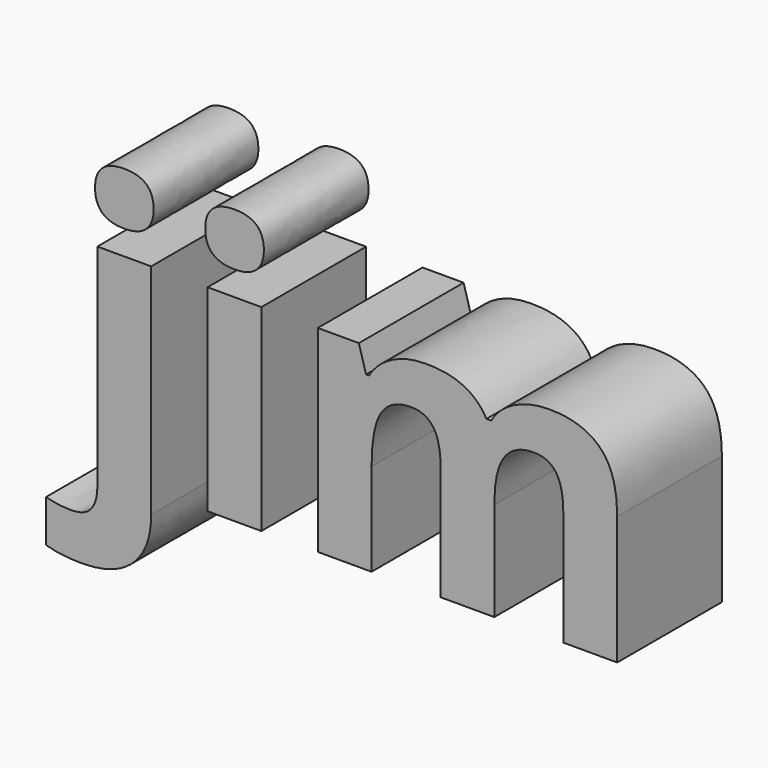
from build123d import *

# Parameters (mm, degrees)
F0_TEXT_SIZE = 23.8288659602
F1_DEPTH     = 8.636


# Not quite as in the source:
# - Text() gives the source's letters only with a copy of the font that has no kerning and outlines rounded to 1/6400 em; it was checked with that copy


with BuildPart() as f1:
    # F0 (on Front) → F1 (new body)
    with BuildSketch(Plane.XZ):
        with Locations((-16.0020012408, 17.4867212772)):
            Text('jim', F0_TEXT_SIZE, font='Open Sans', font_style=FontStyle.BOLD, text_align=(TextAlign.LEFT, TextAlign.BOTTOM))
    extrude(amount=F1_DEPTH)


solid = f1.part
